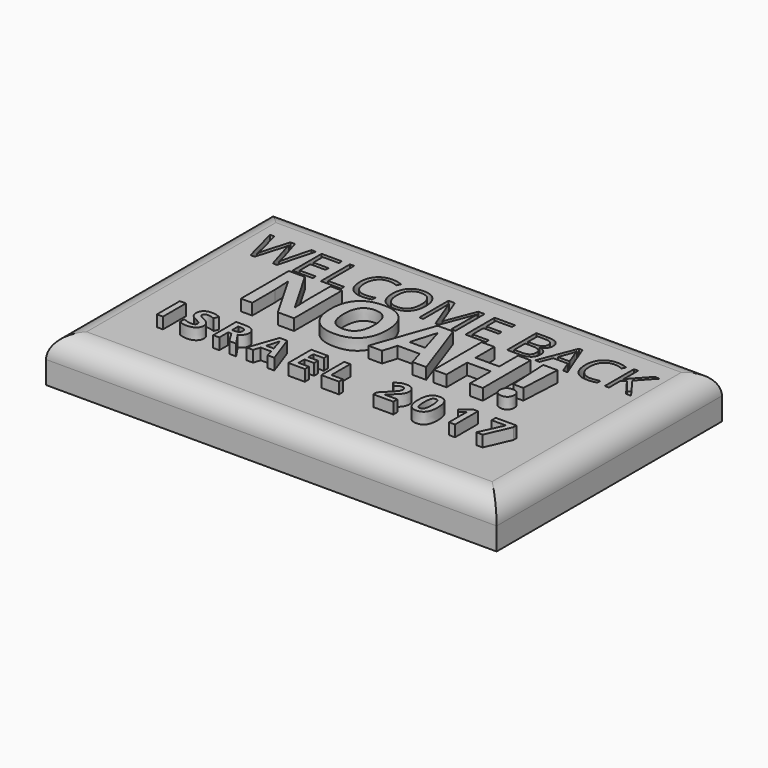
from build123d import *

# Parameters (mm, degrees)
F0_W         = 101.6
F0_H         = 63.5
F1_DEPTH     = 10.16
F2_R         = 5.08
F3_TEXT_SIZE = 11.5160102012
F4_DEPTH     = 2.54
F5_TEXT_SIZE = 18.9164029045
F6_DEPTH     = 2.54
F8_TEXT_SIZE = 9.0599684174
F9_DEPTH     = 2.54


# Not quite as in the source:
# - Text() gives the source's letters only with a copy of the font that has no kerning and outlines rounded to 1/6400 em; it was checked with that copy


with BuildPart() as f1:
    # F0 (on Top) → F1 (new body)
    with BuildSketch(Plane.XY):
        with Locations((-0.6558187306, 15.064227902)):
            Rectangle(F0_W, F0_H)
    extrude(amount=F1_DEPTH)

    # F2
    f2_edges = [f1.edges().sort_by_distance(p)[0] for p in [
        (-51.455819, 15.064228, 10.16),
        (-0.655819, 46.814228, 10.16),
        (50.144181, 15.064228, 10.16),
        (-0.655819, -16.685772, 10.16),
    ]]
    fillet(f2_edges, radius=F2_R)

    # F3 (on face) → F4 (cut)
    with BuildSketch(Plane.XY.offset(10.16)):
        with Locations((-44.4449148021, 29.2480039899)):
            Text('WELCOME BACK', F3_TEXT_SIZE, font='Open Sans', text_align=(TextAlign.LEFT, TextAlign.BOTTOM))
    extrude(amount=-F4_DEPTH, mode=Mode.SUBTRACT)

    # F5 (on face) → F6 (join)
    with BuildSketch(Plane.XY.offset(10.16)):
        with Locations((-31.7296247727, 11.4423874383)):
            Text('NOAH!', F5_TEXT_SIZE, font='Open Sans', font_style=FontStyle.BOLD, text_align=(TextAlign.LEFT, TextAlign.BOTTOM))
    extrude(amount=F6_DEPTH)

    # F8 (on face) → F9 (join)
    with BuildSketch(Plane.XY.offset(10.16)):
        with Locations((-38.6401005089, -2.4855153169)):
            Text('I S R A E L   2 0 1 7', F8_TEXT_SIZE, font='Open Sans', font_style=FontStyle.BOLD, text_align=(TextAlign.LEFT, TextAlign.BOTTOM))
    extrude(amount=F9_DEPTH)


solid = f1.part
